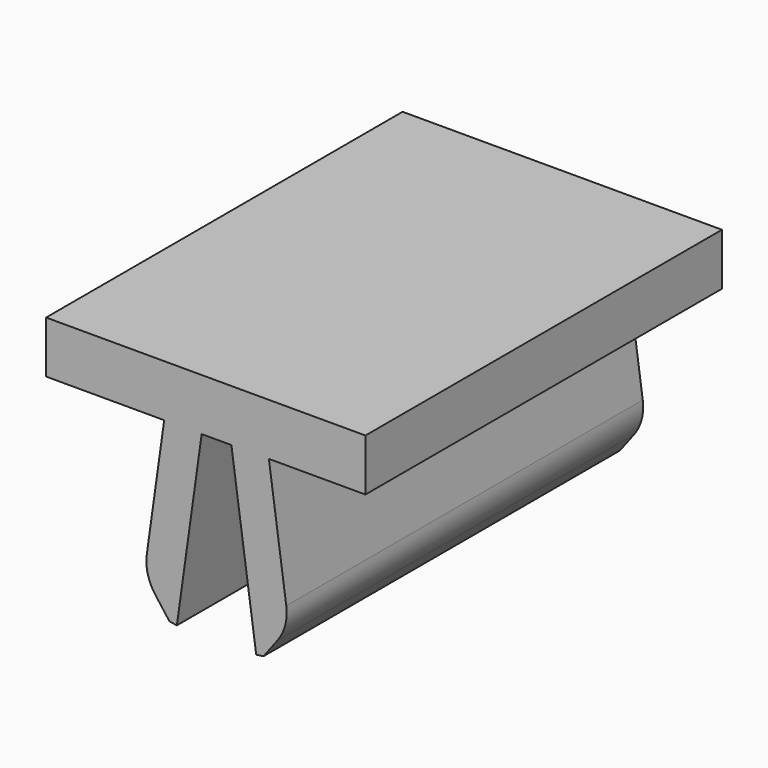
from build123d import *

# Parameters (mm, degrees)
F1_DEPTH = 30
F2_DEPTH = 3.5
F3_DEPTH = 5
F4_SIZE  = 2
F5_R     = 3


# Not quite as in the source:
# - a feature names something its author has since deleted; it is built from what else it names


with BuildPart() as f1:
    # F0 (on Front) → F1 (new body)
    with BuildSketch(Plane.XZ):
        Polygon((5.4754310687, 0), (2.9508621374, 0), (1.3296836853, -11.5352840725), (3.8053538572, -11.8832168249), align=None)
        Polygon((10, 0), (7.4754310687, 0), (9.1455082802, -11.8832168249), (11.6211784521, -11.5352840725), align=None)
        Polygon((0, 3.5), (0, 0), (2.9508621374, 0), (5.4754310687, 0), (7.4754310687, 0), (10, 0), (12.5, 0), (15.5, 0), (20, 0), (20, 3.5), align=None)
    extrude(amount=F1_DEPTH)

    # F2 (cut): a face of the model
    f2_faces = [f1.faces().sort_by_distance(p)[0] for p in [
        (20, -15, 1.75),
    ]]
    extrude(f2_faces, amount=-F2_DEPTH, mode=Mode.SUBTRACT)

    # F3 (add): a face of the model
    f3_faces = [f1.faces().sort_by_distance(p)[0] for p in [
        (0, -15, 1.75),
    ]]
    extrude(f3_faces, amount=F3_DEPTH)

    # F4
    f4_edges = [f1.edges().sort_by_distance(p)[0] for p in [
        (11.621178, -15, -11.535284),
        (1.329684, -15, -11.535284),
    ]]
    chamfer(f4_edges, length=F4_SIZE)

    # F5
    f5_edges = [f1.edges().sort_by_distance(p)[0] for p in [
        (1.60803, -15, -9.554748),
        (11.342832, -15, -9.554748),
    ]]
    fillet(f5_edges, radius=F5_R)


solid = f1.part
